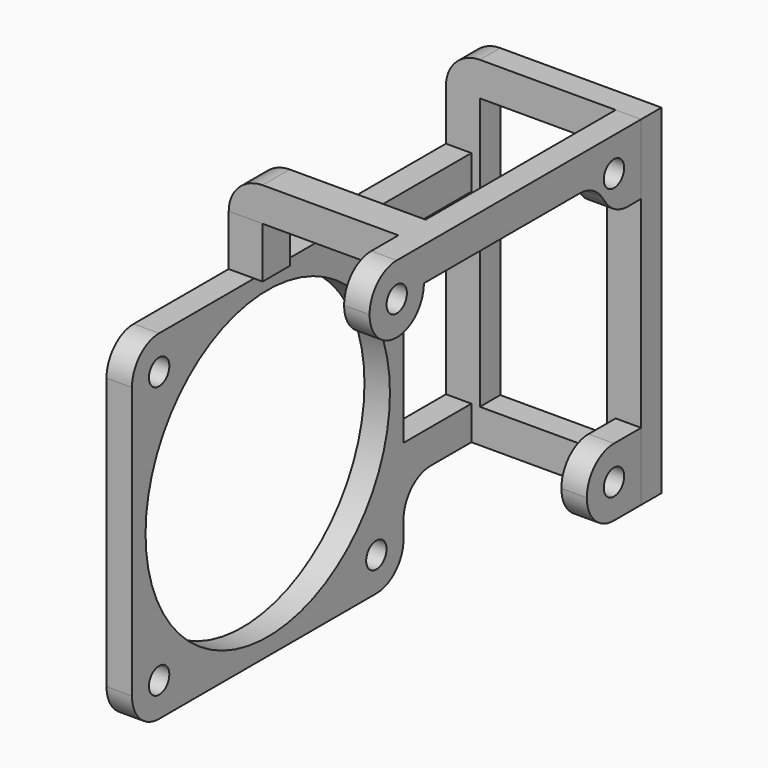
from build123d import *

# Parameters (mm, degrees)
F0_W      = 3
F0_H      = 40
F0_H_2    = 10
F3_DEPTH  = 50
F2_W      = 3
F2_H      = 40
F4_DEPTH  = 40
F1_W      = 23
F1_H      = 3
F5_DEPTH  = 40
F6_R      = 18
F7_DEPTH  = 3
F8_R      = 1.5
F9_DEPTH  = 3
F11_DEPTH = 3
F12_R     = 1.5
F13_DEPTH = 3
F14_W     = 15
F14_H     = 32
F15_DEPTH = 3
F16_W     = 10
F16_H     = 10
F17_DEPTH = 3
F18_W     = 10
F18_H     = 22
F18_W_2   = 50
F18_H_2   = 10
F19_DEPTH = 3
F20_W     = 4
F20_H     = 23.7494786941
F21_DEPTH = 3
F22_R     = 3.99999
F22_2_R   = 3.99999
F23_W     = 4
F23_H     = 4
F24_DEPTH = 20
F25_W     = 4
F25_H     = 4
F26_DEPTH = 6
F27_R     = 3.99999
F27_2_R   = 3.99999


# Not quite as in the source:
# - a fillet or chamfer is up to 0.001 mm smaller than in the source, because OpenCascade refuses the exact size


with BuildPart() as f3:
    # F0 (on Top) → F3 (new body)
    with BuildSketch(Plane.XY):
        with Locations((1.5, 20)):
            Rectangle(F0_W, F0_H)
        with Locations((1.5, 45)):
            Rectangle(F0_W, F0_H_2)
    extrude(amount=-F3_DEPTH)

    # F6 (on face) → F7 (cut)
    with BuildSketch(Plane(origin=(0, 0, 0), x_dir=(0, -1, 0), z_dir=(-1, 0, 0))):
        with Locations((-20, -30)):
            Circle(F6_R)
    extrude(amount=-F7_DEPTH, mode=Mode.SUBTRACT)

    # F8 (on face) → F9 (cut)
    with BuildSketch(Plane(origin=(0, 0, 0), x_dir=(0, -1, 0), z_dir=(-1, 0, 0))):
        with Locations((-4, -14)):
            Circle(F8_R)
        with Locations((-4, -46)):
            Circle(F8_R)
        with Locations((-36, -14)):
            Circle(F8_R)
        with Locations((-36, -46)):
            Circle(F8_R)
    extrude(amount=-F9_DEPTH, mode=Mode.SUBTRACT)

    # F16 (on face) → F17 (cut)
    with BuildSketch(Plane(origin=(0, 0, 0), x_dir=(0, -1, 0), z_dir=(-1, 0, 0))):
        with Locations((-45, -45)):
            Rectangle(F16_W, F16_H)
    extrude(amount=-F17_DEPTH, mode=Mode.SUBTRACT)

    # F18 (on face) → F19 (cut)
    with BuildSketch(Plane(origin=(0, 0, 0), x_dir=(0, -1, 0), z_dir=(-1, 0, 0))):
        with Locations((-45, -25)):
            Rectangle(F18_W, F18_H)
        with Locations((-25, -5)):
            Rectangle(F18_W_2, F18_H_2)
    extrude(amount=-F19_DEPTH, mode=Mode.SUBTRACT)

    # F22#2 (radius 4 in the source; OpenCascade refuses exactly that, so slightly less here)
    f22_2_edges = [f3.edges().sort_by_distance(p)[0] for p in [
        (1.5, 0, -10),
        (1.5, 0, -50),
        (1.5, 40, -50),
        (1.5, 40, -40),
    ]]
    fillet(f22_2_edges, radius=F22_2_R)


with BuildPart() as f4:
    # F2 (on Top) → F4 (new body)
    with BuildSketch(Plane.XY):
        with Locations((21.5, 30)):
            Rectangle(F2_W, F2_H)
    extrude(amount=-F4_DEPTH)

    # F10 (on face) → F11 (cut)
    with BuildSketch(Plane.YZ.offset(23)):
        Polygon((18, -8), (10, -8), (10, -40), (42, -40), (42, -32), (46, -32), (46, -8.2505213059), (43.0126793981, -4), (18, -4), align=None)
    extrude(amount=-F11_DEPTH, mode=Mode.SUBTRACT)

    # F12 (on face) → F13 (cut)
    with BuildSketch(Plane.YZ.offset(23)):
        with Locations((14, -4)):
            Circle(F12_R)
        with Locations((46, -4)):
            Circle(F12_R)
        with Locations((46, -36)):
            Circle(F12_R)
    extrude(amount=-F13_DEPTH, mode=Mode.SUBTRACT)

    # F20 (on face) → F21 (cut)
    with BuildSketch(Plane.YZ.offset(23)):
        with Locations((48, -20.125260653)):
            Rectangle(F20_W, F20_H)
    extrude(amount=-F21_DEPTH, mode=Mode.SUBTRACT)

    # F22 (radius 4 in the source; OpenCascade refuses exactly that, so slightly less here)
    f22_edges = [f4.edges().sort_by_distance(p)[0] for p in [
        (21.5, 10, 0),
        (21.5, 10, -8),
        (21.5, 18, -8),
        (21.5, 43.012679, -4),
        (21.5, 42, -40),
        (21.5, 42, -32),
        (21.5, 46, -8.250521),
    ]]
    fillet(f22_edges, radius=F22_R)

    # F23 (on face) → F24 (join)
    with BuildSketch(Plane(origin=(20, 0, 0), x_dir=(0, -1, 0), z_dir=(-1, 0, 0))):
        with Locations((-20, -2)):
            Rectangle(F23_W, F23_H)
    extrude(amount=F24_DEPTH)

    # F27#2 (radius 4 in the source; OpenCascade refuses exactly that, so slightly less here)
    f27_2_edges = [f4.edges().sort_by_distance(p)[0] for p in [
        (0, 20, 0),
    ]]
    fillet(f27_2_edges, radius=F27_2_R)


with BuildPart() as f5:
    # F1 (on Top) → F5 (new body)
    with BuildSketch(Plane.XY):
        with Locations((11.5, 51.5)):
            Rectangle(F1_W, F1_H)
    extrude(amount=-F5_DEPTH)

    # F14 (on face) → F15 (cut)
    with BuildSketch(Plane(origin=(0, 53, 0), x_dir=(-1, 0, 0), z_dir=(0, 1, 0))):
        with Locations((-11.5, -20)):
            Rectangle(F14_W, F14_H)
    extrude(amount=-F15_DEPTH, mode=Mode.SUBTRACT)

    # F27 (radius 4 in the source; OpenCascade refuses exactly that, so slightly less here)
    f27_edges = [f5.edges().sort_by_distance(p)[0] for p in [
        (0, 51.5, 0),
    ]]
    fillet(f27_edges, radius=F27_R)


with BuildPart() as f26:
    # F25 (on face) → F26 (new body, through all)
    with BuildSketch(Plane(origin=(0, 0, -4), x_dir=(1, 0, 0), z_dir=(0, 0, -1))):
        with Locations((2, -20)):
            Rectangle(F25_W, F25_H)
    extrude(amount=F26_DEPTH)


solid = Compound([f3.part, f4.part, f5.part, f26.part])
